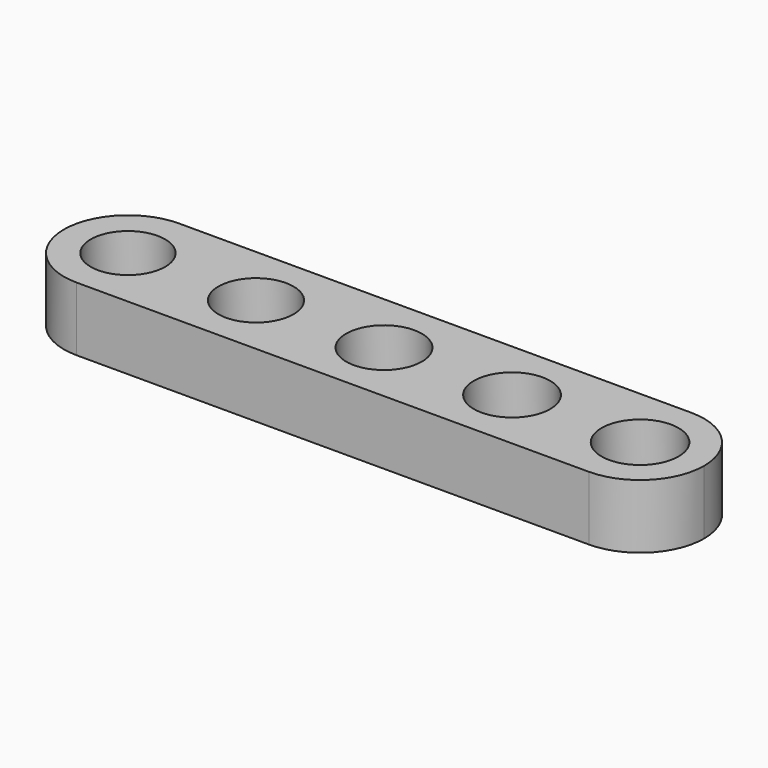
from build123d import *

# Parameters (mm, degrees)
F0_W     = 50
F0_H     = 10
F1_DEPTH = 5
F2_R     = 1.5
F3_DEPTH = 5.001
F5_R     = 4.99999
F4_R     = 2.91
F4_R_2   = 2.935
F4_R_3   = 2.96
F4_R_4   = 2.985
F4_R_5   = 3.01
F6_DEPTH = 3.6


# Not quite as in the source:
# - a fillet or chamfer is up to 0.001 mm smaller than in the source, because OpenCascade refuses the exact size


with BuildPart() as f1:
    # F0 (on Top) → F1 (new body)
    with BuildSketch(Plane.XY):
        with Locations((25, 5)):
            Rectangle(F0_W, F0_H)
    extrude(amount=F1_DEPTH)

    # F2 (on face) → F3 (cut, through all)
    with BuildSketch(Plane(origin=(0, 0, 0), x_dir=(1, 0, 0), z_dir=(0, 0, -1))):
        with Locations((5, -5)):
            Circle(F2_R)
        with Locations((15, -5)):
            Circle(F2_R)
        with Locations((25, -5)):
            Circle(F2_R)
        with Locations((35, -5)):
            Circle(F2_R)
        with Locations((45, -5)):
            Circle(F2_R)
    extrude(amount=-F3_DEPTH, mode=Mode.SUBTRACT)

    # F5 (radius 5 in the source; OpenCascade refuses exactly that, so slightly less here)
    f5_edges = [f1.edges().sort_by_distance(p)[0] for p in [
        (0, 0, 2.5),
        (0, 10, 2.5),
        (50, 0, 2.5),
        (50, 10, 2.5),
    ]]
    fillet(f5_edges, radius=F5_R)

    # F4 (on face) → F6 (cut)
    with BuildSketch(Plane.XY.offset(5)):
        with Locations((5, 5)):
            Circle(F4_R)
        with Locations((15, 5)):
            Circle(F4_R_2)
        with Locations((25, 5)):
            Circle(F4_R_3)
        with Locations((35, 5)):
            Circle(F4_R_4)
        with Locations((45, 5)):
            Circle(F4_R_5)
    extrude(amount=-F6_DEPTH, mode=Mode.SUBTRACT)


solid = f1.part
